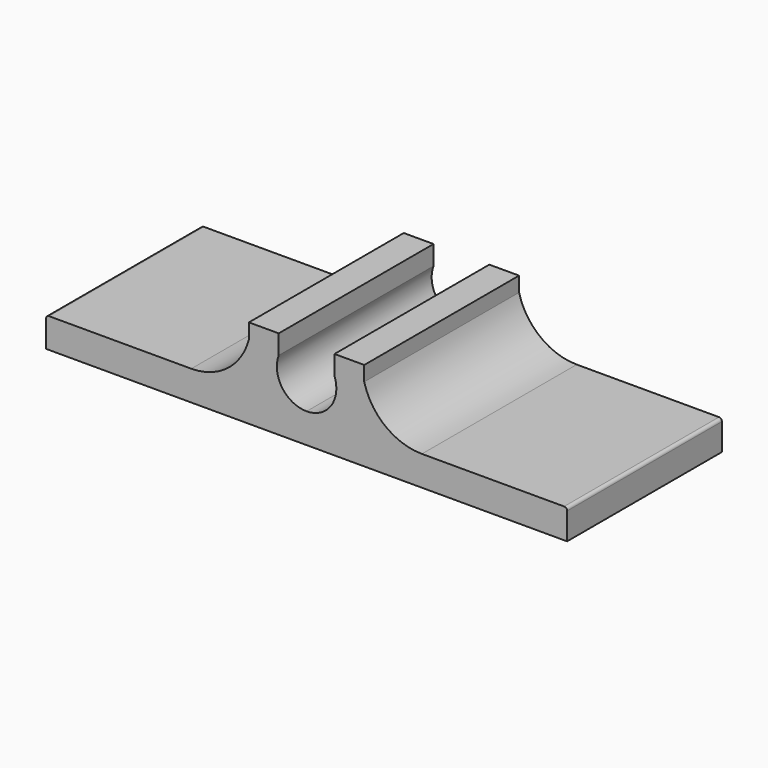
from build123d import *

# Parameters (mm, degrees)
F1_DEPTH    = 13
F2_T1_DEPTH = 13
F3_R        = 0.2


# Not quite as in the source:
# - a fillet or chamfer that OpenCascade refuses, or shapes differently, is made with other operations: its cross-section is extruded or revolved along the edge and cut away or added
# - a feature names something its author has since deleted; it is built from what else it names


with BuildPart() as f1:
    # F0 (on Front) → F1 (new body)
    with BuildSketch(Plane.XZ):
        with BuildLine():
            Line((-3.4641016151, 1), (-17.5, 1))
            Line((-17.5, 1), (-17.5, -1))
            Line((-17.5, -1), (0, -1))
            ThreePointArc((0, -1), (-2, -0.4641016151), (-3.4641016151, 1))
        make_face()
        with BuildLine():
            ThreePointArc((-3.9382737335, 3.7), (-3.9397068673, 2.3081114255), (-3.4641016151, 1))
            Line((-3.4641016151, 1), (7e-09, 1))
            ThreePointArc((7e-09, 1), (-1.6431676705, 1.859824572), (-1.8734993995, 3.7))
            Line((-1.8734993995, 3.7), (-3.9382737335, 3.7))
        make_face()
        with BuildLine():
            Line((7e-09, 1), (-3.4641016151, 1))
            ThreePointArc((-3.4641016151, 1), (-2, -0.4641016151), (0, -1))
            ThreePointArc((0, -1), (2, -0.4641016151), (3.4641016151, 1))
            Line((3.4641016151, 1), (7e-09, 1))
        make_face()
        with BuildLine():
            ThreePointArc((1.8734993995, 3.7), (1.6431676745, 1.8598245778), (7e-09, 1))
            Line((7e-09, 1), (3.4641016151, 1))
            ThreePointArc((3.4641016151, 1), (3.9397068673, 2.3081114255), (3.9382737335, 3.7))
            Line((3.9382737335, 3.7), (1.8734993995, 3.7))
        make_face()
        with BuildLine():
            ThreePointArc((-3.8729833462, 4), (-3.9085079367, 3.8506266565), (-3.9382737335, 3.7))
            Line((-3.9382737335, 3.7), (-1.8734993995, 3.7))
            Line((-1.8734993995, 3.7), (-1.8734993995, 5))
            Line((-1.8734993995, 5), (-3.8729833462, 5))
            Line((-3.8729833462, 5), (-3.8729833462, 4))
        make_face()
        with BuildLine():
            ThreePointArc((3.4641016151, 1), (2, -0.4641016151), (0, -1))
            Line((0, -1), (17.5, -1))
            Line((17.5, -1), (17.5, 1))
            Line((17.5, 1), (3.4641016151, 1))
        make_face()
        with BuildLine():
            Line((1.8734993995, 5), (1.8734993995, 3.7))
            Line((1.8734993995, 3.7), (3.9382737335, 3.7))
            ThreePointArc((3.9382737335, 3.7), (3.9085079367, 3.8506266565), (3.8729833462, 4))
            Line((3.8729833462, 4), (3.8729833462, 5))
            Line((3.8729833462, 5), (1.8734993995, 5))
        make_face()
    extrude(amount=F1_DEPTH)

    # F2: fillet of radius 4 on 2 edges, made by hand

    # F2_s2 → F2_t1 (join)
    with BuildSketch(Plane.XZ):
        with BuildLine():
            ThreePointArc((-7.7459666924, 1), (-5.2964769496, 1.8377223398), (-3.8729833462, 4))
            ThreePointArc((-3.8729833462, 4), (-3.9633576589, 2.4598184865), (-3.4641016151, 1))
            Line((-3.4641016151, 1), (-7.7459666924, 1))
        make_face()
        with BuildLine():
            ThreePointArc((7.7459666924, 1), (5.2964769496, 1.8377223398), (3.8729833462, 4))
            ThreePointArc((3.8729833462, 4), (3.9633576589, 2.4598184865), (3.4641016151, 1))
            Line((3.4641016151, 1), (7.7459666924, 1))
        make_face()
    extrude(amount=F2_T1_DEPTH)

    # F3
    f3_edges = [f1.edges().sort_by_distance(p)[0] for p in [
        (-17.5, -6.5, 1),
        (17.5, -6.5, 1),
    ]]
    fillet(f3_edges, radius=F3_R)


solid = f1.part
